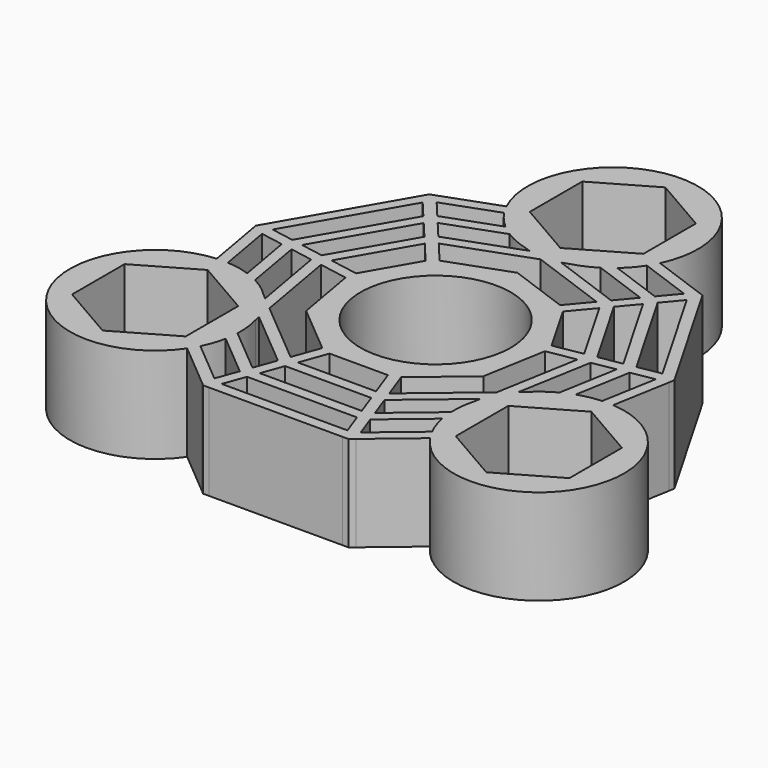
from build123d import *

# Parameters (mm, degrees)
F0_R     = 12.5
F1_DEPTH = 14
F0_R_2   = 11.025
F2_COUNT = 3
F4_DEPTH = 14
F5_COUNT = 3


# Not quite as in the source:
# - a feature names something its author has since deleted; it is built from what else it names


with BuildPart() as f1:
    # F0 (on Top) → F1 (new body)
    with BuildSketch(Plane.XY):
        with Locations((0, 32.5)):
            Circle(F0_R)
        Polygon((8.3354945114, 37.3125), (8.3354945114, 27.6875), (0, 22.875), (-8.3354945114, 27.6875), (-8.3354945114, 37.3125), (0, 42.125), align=None, mode=Mode.SUBTRACT)
    extrude(amount=F1_DEPTH)


with BuildPart() as f1b:
    # F0 (on Top) → F1, piece 2 (new body)
    with BuildSketch(Plane.XY):
        Polygon((9.6418141453, 11.4906666468), (0, 15), (-9.6418141453, 11.4906666468), (-14.7721162952, 2.604722665), (-12.9903810568, -7.5), (-5.1303021499, -14.0953893118), (5.1303021499, -14.0953893118), (12.9903810568, -7.5), (14.7721162952, 2.604722665), align=None)
        Circle(F0_R_2, mode=Mode.SUBTRACT)
    extrude(amount=F1_DEPTH)


with BuildPart() as f2_1:
    # F2: instance of F1
    add(f1.part.rotate(Axis((0, 0, 0), (0, 0, -1)), 1 * 360 / F2_COUNT))


with BuildPart() as f2_2:
    # F2: instance of F1
    add(f1.part.rotate(Axis((0, 0, 0), (0, 0, -1)), 2 * 360 / F2_COUNT))


with BuildPart() as f1_1:
    add(f1.part)

    add(f1b.part)  # F4 merges F1b

    add(f2_2.part)  # F4 merges F2_2
    # F3 (on Top) → F4 (join, through all)
    with BuildSketch(Plane.XY):
        Polygon((-14.3464451862, 3.3420066531), (-18.5384872699, 4.0811767767), (-18.9641583789, 3.3438927886), (-18.8163243541, 2.5054843719), (-14.6242822705, 1.7663142483), (-14.7721162952, 2.604722665), align=None)
        Polygon((-8.8418141453, 11.7818428342), (-11.5779752919, 15.0426727106), (-12.3779752919, 14.7514965232), (-12.8036464009, 14.0142125351), (-10.0674852543, 10.7533826587), (-9.6418141453, 11.4906666468), align=None)
        Polygon((-18.9641583789, 3.3438927886), (-18.5384872699, 4.0811767767), (-20.2153041033, 4.3768448262), (-20.6409752123, 3.6395608381), (-20.4931411876, 2.8011524213), (-18.8163243541, 2.5054843719), align=None)
        Polygon((-12.3779752919, 14.7514965232), (-11.5779752919, 15.0426727106), (-12.6724397505, 16.3470046611), (-13.4724397505, 16.0558284737), (-13.8981108595, 15.3185444856), (-12.8036464009, 14.0142125351), align=None)
        Polygon((-13.4724397505, 16.0558284737), (-12.6724397505, 16.3470046611), (-14.8613686678, 18.9556685622), (-15.6613686678, 18.6644923748), (-16.0870397768, 17.9272083867), (-13.8981108595, 15.3185444856), align=None)
        Polygon((-20.6409752123, 3.6395608381), (-20.2153041033, 4.3768448262), (-23.5689377703, 4.968180925), (-23.9946088793, 4.230896937), (-23.8467748545, 3.3924885202), (-20.4931411876, 2.8011524213), align=None)
        Polygon((-23.5689377703, 4.968180925), (-25.2457546037, 5.2638489745), (-25.6714257127, 4.5265649864), (-25.523591688, 3.6881565697), (-23.8467748545, 3.3924885202), (-23.9946088793, 4.230896937), align=None)
        Polygon((-14.8613686678, 18.9556685622), (-15.9558331265, 20.2600005128), (-16.7558331265, 19.9688243254), (-17.1815042355, 19.2315403373), (-16.0870397768, 17.9272083867), (-15.6613686678, 18.6644923748), align=None)
        Polygon((-15.9558331265, 20.2600005128), (-18.1447620438, 22.8686644139), (-18.9447620438, 22.5774882265), (-19.3704331527, 21.8402042384), (-17.1815042355, 19.2315403373), (-16.7558331265, 19.9688243254), align=None)
        Polygon((-25.2457546037, 5.2638489745), (-28.5993882707, 5.8551850734), (-29.0250593797, 5.1179010853), (-28.8772253549, 4.2794926686), (-25.523591688, 3.6881565697), (-25.6714257127, 4.5265649864), align=None)
        Polygon((-28.5993882707, 5.8551850734), (-30.2762051041, 6.1508531228), (-30.7018762131, 5.4135691347), (-30.5540421884, 4.575160718), (-28.8772253549, 4.2794926686), (-29.0250593797, 5.1179010853), align=None)
        Polygon((-18.1447620438, 22.8686644139), (-19.2392265024, 24.1729963645), (-20.0392265024, 23.881820177), (-20.4648976114, 23.144536189), (-19.3704331527, 21.8402042384), (-18.9447620438, 22.5774882265), align=None)
        with BuildLine():
            ThreePointArc((-10.4650421032, 25.6638538798), (-10.8865068143, 26.3572018279), (-11.262100915, 27.0764326333))
            Line((-11.262100915, 27.0764326333), (-19.2392265024, 24.1729963645))
            Line((-19.2392265024, 24.1729963645), (-18.1447620438, 22.8686644139))
            Line((-18.1447620438, 22.8686644139), (-10.4650421032, 25.6638538798))
        make_face()
        Polygon((-19.3704331527, 21.8402042384), (-20.4648976114, 23.144536189), (-30.2762051041, 6.1508531228), (-28.5993882707, 5.8551850734), align=None)
        Polygon((-16.0870397768, 17.9272083867), (-17.1815042355, 19.2315403373), (-25.2457546037, 5.2638489745), (-23.5689377703, 4.968180925), align=None)
        with BuildLine():
            ThreePointArc((-6.6788350915, 21.9338672249), (-7.4683996582, 22.4763775737), (-8.2140988038, 23.0777613678))
            Line((-8.2140988038, 23.0777613678), (-15.9558331265, 20.2600005128))
            Line((-15.9558331265, 20.2600005128), (-14.8613686678, 18.9556685622))
            Line((-14.8613686678, 18.9556685622), (-6.6788350915, 21.9338672249))
        make_face()
        with BuildLine():
            Line((-11.5779752919, 15.0426727106), (3.1518577067, 20.4038934778))
            ThreePointArc((3.1518577067, 20.4038934778), (0.5214979159, 20.0108831408), (-2.1324694589, 20.1832401173))
            Line((-2.1324694589, 20.1832401173), (-12.6724397505, 16.3470046611))
            Line((-12.6724397505, 16.3470046611), (-11.5779752919, 15.0426727106))
        make_face()
        Polygon((-18.5384872699, 4.0811767767), (-12.8036464009, 14.0142125351), (-13.8981108595, 15.3185444856), (-20.2153041033, 4.3768448262), align=None)
        with BuildLine():
            Line((-28.8772253549, 4.2794926686), (-30.5540421884, 4.575160718))
            Line((-30.5540421884, 4.575160718), (-29.0799289618, -3.7849508243))
            ThreePointArc((-29.0799289618, -3.7849508243), (-28.2692597628, -3.7506094543), (-27.4580704705, -3.7689346268))
            Line((-27.4580704705, -3.7689346268), (-28.8772253549, 4.2794926686))
        make_face()
        with BuildLine():
            Line((-23.8467748545, 3.3924885202), (-25.523591688, 3.6881565697))
            Line((-25.523591688, 3.6881565697), (-24.0929770089, -4.4252624506))
            ThreePointArc((-24.0929770089, -4.4252624506), (-23.199313793, -4.7703649572), (-22.3347037658, -5.1828927555))
            Line((-22.3347037658, -5.1828927555), (-23.8467748545, 3.3924885202))
        make_face()
        with BuildLine():
            Line((-16.0943612345, -12.931535582), (-18.8163243541, 2.5054843719))
            Line((-18.8163243541, 2.5054843719), (-20.4931411876, 2.8011524213))
            Line((-20.4931411876, 2.8011524213), (-18.5454334017, -8.2448473345))
            ThreePointArc((-18.5454334017, -8.2448473345), (-17.0691841941, -10.4570720136), (-16.0943612345, -12.931535582))
        make_face()
    extrude(amount=F4_DEPTH)



with BuildPart() as f1_2:
    add(f1_1.part)

    add(f2_1.part)  # F5 merges F2_1
    # F5: F1 ×3 about axis
    f5_axis = Axis((0, 0, 0), (0, 0, -1))
    for i in range(1, F5_COUNT):
        add(f1_1.part.rotate(f5_axis, i * 360 / F5_COUNT))


solid = f1_2.part
